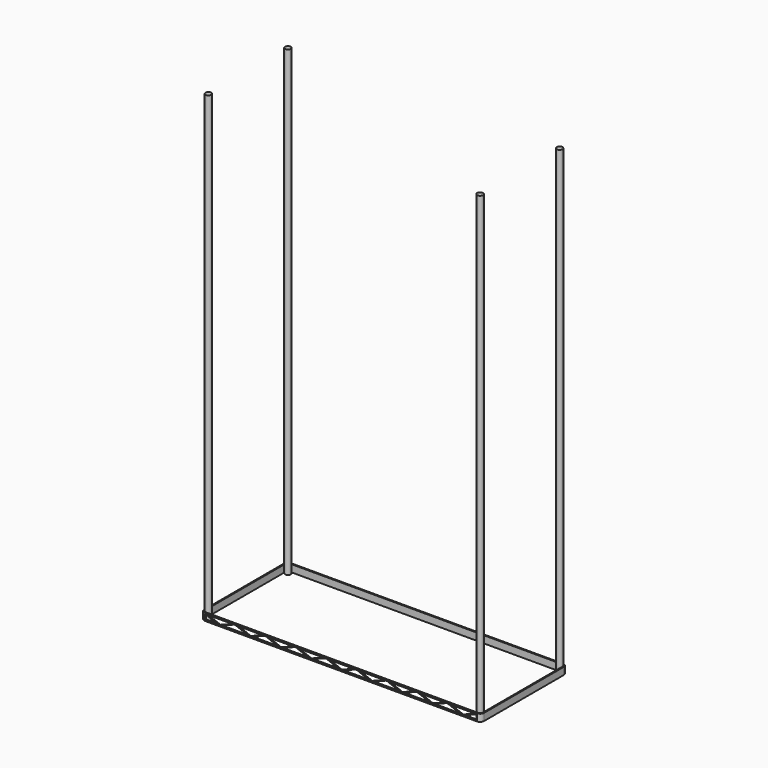
from build123d import *

# Parameters (mm, degrees)
F1_DEPTH = 31
F2_R     = 12.75
F3_DEPTH = 2000
F5_DEPTH = 25


# Not quite as in the source:
# - ends of sketch curves that miss each other by under 0.0002 mm in the source are joined


with BuildPart() as f1:
    # F0 (on Top) → F1 (new body)
    with BuildSketch(Plane.XY):
        with BuildLine():
            Line((-4.9999998882, 442.5), (-4.9999998882, 12.5))
            ThreePointArc((-4.9999998882, 12.5), (0.1256313292, 0.1256313292), (12.5, -5))
            Line((12.5, -5), (1187.5, -5))
            ThreePointArc((1187.5, -5), (1199.8743686708, 0.1256313292), (1205, 12.5))
            Line((1205, 12.5), (1205, 442.5))
            ThreePointArc((1205, 442.5), (1199.8743686708, 454.8743686708), (1187.5, 460))
            Line((1187.5, 460), (12.5, 460.0000083447))
            ThreePointArc((12.5, 460.0000083447), (0.1256313292, 454.8743686708), (-4.9999998882, 442.5))
        make_face()
        with BuildLine():
            Line((1187.5, 0), (12.5, 0))
            ThreePointArc((12.5, 0), (3.6611652352, 3.6611652352), (0, 12.5))
            Line((0, 12.5), (0, 442.5))
            ThreePointArc((0, 442.5), (3.6611652352, 451.3388347648), (12.5, 455))
            Line((12.5, 455), (1187.5, 455))
            ThreePointArc((1187.5, 455), (1196.3388347648, 451.3388347648), (1200, 442.5))
            Line((1200, 442.5), (1200, 12.5))
            ThreePointArc((1200, 12.5), (1196.3388347648, 3.6611652352), (1187.5, 0))
        make_face(mode=Mode.SUBTRACT)
    extrude(amount=F1_DEPTH)

    # F2 (on Top) → F3 (join)
    with BuildSketch(Plane.XY):
        with Locations((12.7221517224, 12.6146673983)):
            Circle(F2_R)
        with Locations((12.7221517224, 442.3853326017)):
            Circle(F2_R)
        with Locations((1187.2778482776, 442.3853326017)):
            Circle(F2_R)
        with Locations((1187.2778482776, 12.6146673983)):
            Circle(F2_R)
    extrude(amount=F3_DEPTH)

    # F4 (on Front) → F5 (cut)
    with BuildSketch(Plane.XZ):
        Polygon((1187.5, 26.9953021277), (1128.762, 4), (1187.5, 4), align=None)
        Polygon((1066.012, 27), (1124.762, 4), (1183.512, 27), align=None)
        Polygon((1056.323, 27), (997.573, 4), (1120.762, 4), (1062.012, 27), align=None)
        Polygon((934.823, 27), (993.573, 4), (1052.323, 27), align=None)
        Polygon((925.134, 27), (866.384, 4), (989.573, 4), (930.823, 27), align=None)
        Polygon((803.634, 27), (862.384, 4), (921.134, 27), align=None)
        Polygon((793.945, 27), (735.195, 4), (858.384, 4), (799.634, 27), align=None)
        Polygon((672.445, 27), (731.195, 4), (789.945, 27), align=None)
        Polygon((662.756, 27), (604.006, 4), (727.195, 4), (668.445, 27), align=None)
        Polygon((541.256, 27), (600.006, 4), (658.756, 27), align=None)
        Polygon((531.567, 27), (472.817, 4), (596.006, 4), (537.256, 27), align=None)
        Polygon((410.067, 27), (468.817, 4), (527.567, 27), align=None)
        Polygon((400.378, 27), (341.628, 4), (464.817, 4), (406.067, 27), align=None)
        Polygon((278.878, 27), (337.628, 4), (396.378, 27), align=None)
        Polygon((269.189, 27), (210.439, 4), (333.628, 4), (274.878, 27), align=None)
        Polygon((265.189, 27), (147.689, 27), (206.439, 4), align=None)
        Polygon((143.689, 27), (138, 27), (79.25, 4), (202.439, 4), align=None)
        Polygon((134, 27), (16.5, 27), (75.25, 4), align=None)
        Polygon((71.25, 4), (12.5, 27), (12.5, 4), align=None)
    extrude(amount=F5_DEPTH, mode=Mode.SUBTRACT)


solid = f1.part
